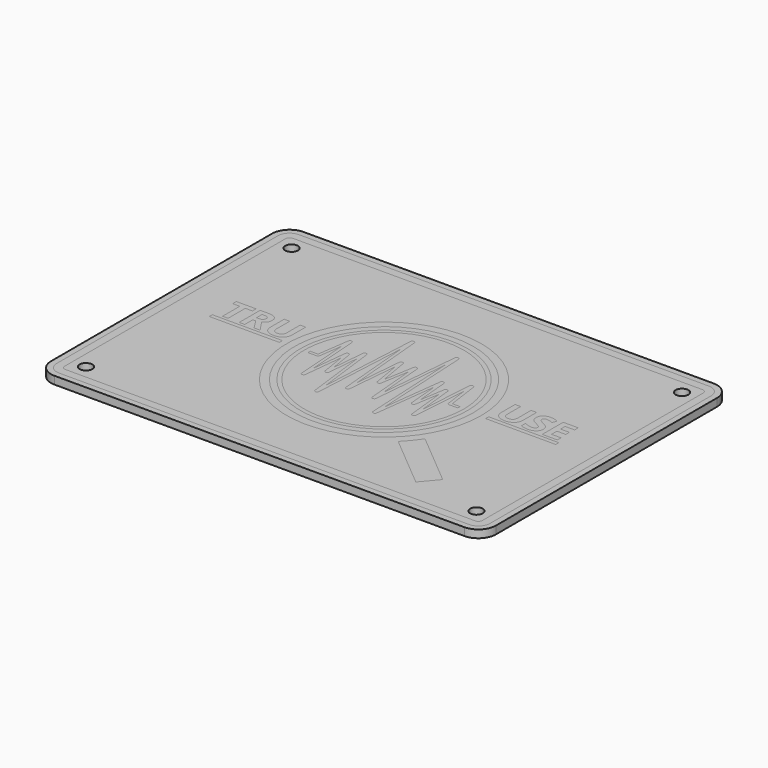
from build123d import *

# Parameters (mm, degrees)
F0_W           = 114.3
F0_H           = 2
F1_DEPTH       = 40
F3_R           = 25
F3_R_2         = 23
F4_DEPTH       = 1
F3_W           = 18
F3_H           = 1
F5_R           = 21.5
F5_R_2         = 20.5
F6_DEPTH       = 1
F8_DEPTH       = 1
F9_TEXT_SIZE   = 9.4236111111
F10_DEPTH      = 1
F12_DEPTH      = 1
F14_DEPTH      = 1
F15_R          = 4.5
F22_R          = 1.632
F23_DEPTH      = 1.0010001
F23_DEPTH_BACK = 1.001


# Not quite as in the source:
# - Text() gives the source's letters only with a copy of the font that has no kerning and outlines rounded to 1/6400 em; it was checked with that copy


with BuildPart() as f1:
    # F0 (on Front) → F1 (new body, symmetric)
    with BuildSketch(Plane.XZ):
        with Locations((0, 1)):
            Rectangle(F0_W, F0_H)
    extrude(amount=F1_DEPTH, both=True)

    # F15
    f15_edges = [f1.edges().sort_by_distance(p)[0] for p in [
        (57.15, 40, 1),
        (57.15, -40, 1),
        (-57.15, -40, 1),
        (-57.15, 40, 1),
    ]]
    fillet(f15_edges, radius=F15_R)


with BuildPart() as f4:
    # F3 (on offset) → F4 (new body)
    with BuildSketch(Plane.XY.offset(1)):
        Circle(F3_R)
        Circle(F3_R_2, mode=Mode.SUBTRACT)
    extrude(amount=F4_DEPTH)


with BuildPart() as f4b:
    # F3 (on offset) → F4, piece 2 (new body)
    with BuildSketch(Plane.XY.offset(1)):
        with Locations((-35.495282599, 0)):
            Rectangle(F3_W, F3_H)
    extrude(amount=F4_DEPTH)


with BuildPart() as f4c:
    # F3 (on offset) → F4, piece 3 (new body)
    with BuildSketch(Plane.XY.offset(1)):
        with Locations((35.495282599, 0)):
            Rectangle(F3_W, F3_H)
    extrude(amount=F4_DEPTH)


with BuildPart() as f6:
    # F5 (on offset) → F6 (new body)
    with BuildSketch(Plane.XY.offset(1)):
        Circle(F5_R)
        Circle(F5_R_2, mode=Mode.SUBTRACT)
    extrude(amount=F6_DEPTH)


with BuildPart() as f8:
    # F7 (on offset) → F8 (new body)
    with BuildSketch(Plane.XY.offset(1)):
        with BuildLine():
            ThreePointArc((22.4888517639, -14.9416045437), (20.8499880973, -17.154532822), (18.9942466389, -19.1890227635))
            Line((18.9942466389, -19.1890227635), (32.7830466151, -30.7591997379))
            Line((32.7830466151, -30.7591997379), (36.3183784684, -26.5459553007))
            Line((36.3183784684, -26.5459553007), (22.4888517639, -14.9416045437))
        make_face()
    extrude(amount=F8_DEPTH)


with BuildPart() as f10:
    # F9 (on offset) → F10 (new body)
    with BuildSketch(Plane.XY.offset(1)):
        with Locations((-44.4958522604, 1.25)):
            Text('TRU', F9_TEXT_SIZE, font='Open Sans', font_style=FontStyle.BOLD, text_align=(TextAlign.LEFT, TextAlign.BOTTOM))
        with Locations((26.495282599, 1.25)):
            Text('USE', F9_TEXT_SIZE, font='Open Sans', font_style=FontStyle.BOLD, text_align=(TextAlign.LEFT, TextAlign.BOTTOM))
    extrude(amount=F10_DEPTH)


with BuildPart() as f12:
    # F11 (on offset) → F12 (new body)
    with BuildSketch(Plane.XY.offset(1)):
        with BuildLine():
            ThreePointArc((55.65, 35.5), (54.7713203436, 37.6213203436), (52.65, 38.5))
            Line((52.65, 38.5), (-52.65, 38.5))
            ThreePointArc((-52.65, 38.5), (-54.7713203436, 37.6213203436), (-55.65, 35.5))
            Line((-55.65, 35.5), (-55.65, -35.5))
            ThreePointArc((-55.65, -35.5), (-54.7713203436, -37.6213203436), (-52.65, -38.5))
            Line((-52.65, -38.5), (52.65, -38.5))
            ThreePointArc((52.65, -38.5), (54.7713203436, -37.6213203436), (55.65, -35.5))
            Line((55.65, -35.5), (55.65, 35.5))
        make_face()
        with BuildLine():
            Line((-52.65, 36.5), (52.65, 36.5))
            ThreePointArc((52.65, 36.5), (53.3571067812, 36.2071067812), (53.65, 35.5))
            Line((53.65, 35.5), (53.65, -35.5))
            ThreePointArc((53.65, -35.5), (53.3571067812, -36.2071067812), (52.65, -36.5))
            Line((52.65, -36.5), (-52.65, -36.5))
            ThreePointArc((-52.65, -36.5), (-53.3571067812, -36.2071067812), (-53.65, -35.5))
            Line((-53.65, -35.5), (-53.65, 35.5))
            ThreePointArc((-53.65, 35.5), (-53.3571067812, 36.2071067812), (-52.65, 36.5))
        make_face(mode=Mode.SUBTRACT)
    extrude(amount=F12_DEPTH)


with BuildPart() as f14:
    # F13 (on offset) → F14 (new body)
    with BuildSketch(Plane.XY.offset(1)):
        with BuildLine():
            Line((-19.246, -0.375), (-17.0286783155, -0.375))
            ThreePointArc((-17.0286783155, -0.375), (-16.7006488011, -0.2523547901), (-16.5335442812, 0.0554134495))
            Line((-16.5335442812, 0.0554134495), (-15.6759470089, 6.1575351145))
            Line((-15.6759470089, 6.1575351145), (-14.6795016964, -8.0922967435))
            ThreePointArc((-14.6795016964, -8.0922967435), (-14.1894458745, -8.5573423542), (-13.6834587235, -8.1096827382))
            Line((-13.6834587235, -8.1096827382), (-12.6175820055, 2.0314568202))
            Line((-12.6175820055, 2.0314568202), (-11.5985237765, -4.4026236167))
            ThreePointArc((-11.5985237765, -4.4026236167), (-11.0872298579, -4.8241017977), (-10.6065822572, -4.3679842556))
            Line((-10.6065822572, -4.3679842556), (-9.893414205, 3.7835638814))
            Line((-9.893414205, 3.7835638814), (-7.9235980217, -12.2593015149))
            ThreePointArc((-7.9235980217, -12.2593015149), (-7.4098751976, -12.6980622567), (-6.9280101785, -12.2245348213))
            Line((-6.9280101785, -12.2245348213), (-5.6264531843, 12.6106520923))
            Line((-5.6264531843, 12.6106520923), (-3.8774286777, -7.3807894974))
            ThreePointArc((-3.8774286777, -7.3807894974), (-3.3793313286, -7.837211626), (-2.8812339796, -7.3807894974))
            Line((-2.8812339796, -7.3807894974), (-1.7329588751, 5.7440550049))
            Line((-1.7329588751, 5.7440550049), (-0.4928914516, -1.5313175141))
            ThreePointArc((-0.4928914516, -1.5313175141), (0, -1.9473055091), (0.4928914516, -1.5313175141))
            Line((0.4928914516, -1.5313175141), (1.7329588751, 5.7440550049))
            Line((1.7329588751, 5.7440550049), (2.8812339796, -7.3807894974))
            ThreePointArc((2.8812339796, -7.3807894974), (3.3793313286, -7.837211626), (3.8774286777, -7.3807894974))
            Line((3.8774286777, -7.3807894974), (5.6264531843, 12.6106520923))
            Line((5.6264531843, 12.6106520923), (6.9280101785, -12.2245348213))
            ThreePointArc((6.9280101785, -12.2245348213), (7.4098751976, -12.6980622567), (7.9235980217, -12.2593015149))
            Line((7.9235980217, -12.2593015149), (9.893414205, 3.7835638814))
            Line((9.893414205, 3.7835638814), (10.6065822572, -4.3679842556))
            ThreePointArc((10.6065822572, -4.3679842556), (11.0872298579, -4.8241017977), (11.5985237765, -4.4026236167))
            Line((11.5985237765, -4.4026236167), (12.6175820055, 2.0314568202))
            Line((12.6175820055, 2.0314568202), (13.6834587235, -8.1096827382))
            ThreePointArc((13.6834587235, -8.1096827382), (14.1894458745, -8.5573423542), (14.6795016964, -8.0922967435))
            Line((14.6795016964, -8.0922967435), (15.6759470089, 6.1575351145))
            Line((15.6759470089, 6.1575351145), (16.5335442812, 0.0554134495))
            ThreePointArc((16.5335442812, 0.0554134495), (16.7006488011, -0.2523547901), (17.0286783155, -0.375))
            Line((17.0286783155, -0.375), (19.246, -0.375))
            Line((19.246, -0.375), (19.246, 0.375))
            Line((19.246, 0.375), (17.246, 0.375))
            Line((17.246, 0.375), (16.0876121593, 8.6173577686))
            ThreePointArc((16.0876121593, 8.6173577686), (15.5750283766, 9.0474666316), (15.0936960998, 8.582649455))
            Line((15.0936960998, 8.582649455), (14.1306586945, -5.1894270707))
            Line((14.1306586945, -5.1894270707), (13.1649803009, 3.9983891119))
            ThreePointArc((13.1649803009, 3.9983891119), (12.6808078273, 4.4459535427), (12.1738751829, 4.0243421128))
            Line((12.1738751829, 4.0243421128), (11.1762716402, -2.2742787658))
            Line((11.1762716402, -2.2742787658), (10.4332523534, 6.2184705447))
            ThreePointArc((10.4332523534, 6.2184705447), (9.9438812076, 6.6748165209), (9.4388819285, 6.235827345))
            Line((9.4388819285, 6.235827345), (7.5274316503, -9.3316859008))
            Line((7.5274316503, -9.3316859008), (6.1883155745, 16.2201709822))
            ThreePointArc((6.1883155745, 16.2201709822), (5.6977270103, 16.6939268516), (5.1909034581, 16.2375808754))
            Line((5.1909034581, 16.2375808754), (3.3793313286, -4.4687833146))
            Line((3.3793313286, -4.4687833146), (2.3108705373, 7.7437794136))
            ThreePointArc((2.3108705373, 7.7437794136), (1.8331571313, 8.1997858643), (1.3198817367, 7.7842135473))
            Line((1.3198817367, 7.7842135473), (0, 0.0405770859))
            Line((0, 0.0405770859), (-1.3198817367, 7.7842135473))
            ThreePointArc((-1.3198817367, 7.7842135473), (-1.8331571313, 8.1997858643), (-2.3108705373, 7.7437794136))
            Line((-2.3108705373, 7.7437794136), (-3.3793313286, -4.4687833146))
            Line((-3.3793313286, -4.4687833146), (-5.1909034581, 16.2375808754))
            ThreePointArc((-5.1909034581, 16.2375808754), (-5.6977270103, 16.6939268516), (-6.1883155745, 16.2201709822))
            Line((-6.1883155745, 16.2201709822), (-7.5274316503, -9.3316859008))
            Line((-7.5274316503, -9.3316859008), (-9.4388819285, 6.235827345))
            ThreePointArc((-9.4388819285, 6.235827345), (-9.9438812076, 6.6748165209), (-10.4332523534, 6.2184705447))
            Line((-10.4332523534, 6.2184705447), (-11.1762716402, -2.2742787658))
            Line((-11.1762716402, -2.2742787658), (-12.1738751829, 4.0243421128))
            ThreePointArc((-12.1738751829, 4.0243421128), (-12.6808078273, 4.4459535427), (-13.1649803009, 3.9983891119))
            Line((-13.1649803009, 3.9983891119), (-14.1306586945, -5.1894270707))
            Line((-14.1306586945, -5.1894270707), (-15.0936960998, 8.582649455))
            ThreePointArc((-15.0936960998, 8.582649455), (-15.5750283766, 9.0474666316), (-16.0876121593, 8.6173577686))
            Line((-16.0876121593, 8.6173577686), (-17.246, 0.375))
            Line((-17.246, 0.375), (-19.246, 0.375))
            Line((-19.246, 0.375), (-19.246, -0.375))
        make_face()
    extrude(amount=F14_DEPTH)


with BuildPart() as f1_1:
    add(f1.part)

    # F16: cut F14
    add(f14.part, mode=Mode.SUBTRACT)

    # F17: cut F4, F4b, F4c
    add(f4.part, mode=Mode.SUBTRACT)
    add(f4b.part, mode=Mode.SUBTRACT)
    add(f4c.part, mode=Mode.SUBTRACT)

    # F18: cut F6
    add(f6.part, mode=Mode.SUBTRACT)

    # F19: cut F8
    add(f8.part, mode=Mode.SUBTRACT)

    # F20: cut F10
    add(f10.part, mode=Mode.SUBTRACT)

    # F21: cut F12
    add(f12.part, mode=Mode.SUBTRACT)

    # F22 (on offset) → F23 (cut, two sides)
    with BuildSketch(Plane.XY.offset(1)) as f23_sk:
        with Locations((-50.15, 33)):
            Circle(F22_R)
        with Locations((50.15, 33)):
            Circle(F22_R)
        with Locations((-50.15, -33)):
            Circle(F22_R)
        with Locations((50.15, -33)):
            Circle(F22_R)
    extrude(amount=F23_DEPTH, mode=Mode.SUBTRACT)
    extrude(f23_sk.sketch, amount=-F23_DEPTH_BACK, mode=Mode.SUBTRACT)


solid = Compound([f4.part, f4b.part, f4c.part, f6.part, f8.part, f10.part, f12.part, f14.part, f1_1.part])
